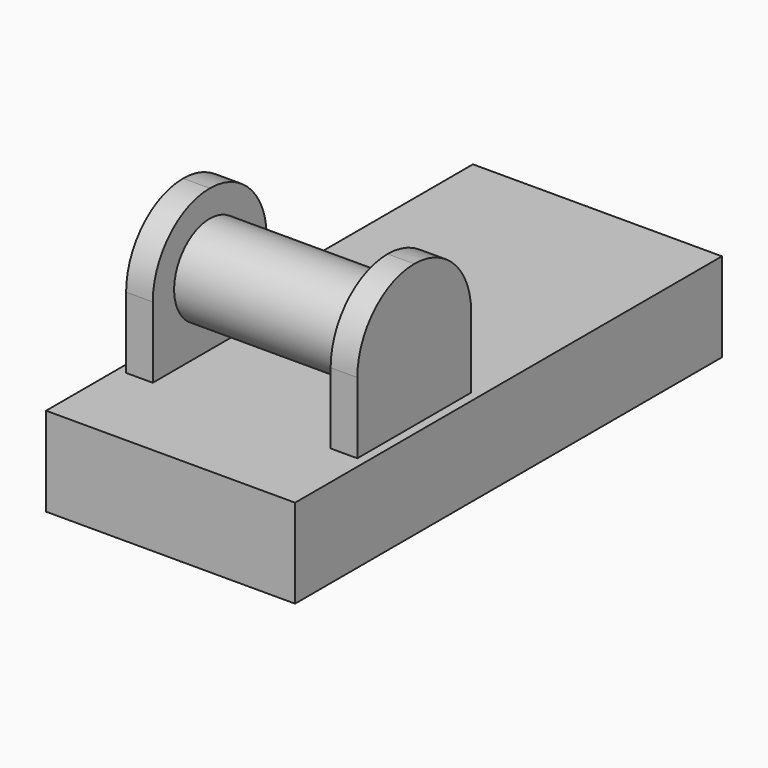
from build123d import *

# Parameters (mm, degrees)
F1_DEPTH = 30
F3_W     = 1.5
F3_H     = 8
F4_DEPTH = 8
F5_R     = 2.5
F6_DEPTH = 13
F7_R     = 3.99999


# Not quite as in the source:
# - a fillet or chamfer is up to 0.001 mm smaller than in the source, because OpenCascade refuses the exact size


with BuildPart() as f1:
    # F0 (on Front) → F1 (new body)
    with BuildSketch(Plane.XZ):
        Polygon((-14, 0), (0, 0), (0, 5), (-0.5, 5), (-2, 5), (-12, 5), (-13.5, 5), (-14, 5), align=None)
    extrude(amount=F1_DEPTH)

    # F3 (on offset) → F4 (join)
    with BuildSketch(Plane.XZ.offset(25)):
        with Locations((-12.75, 9)):
            Rectangle(F3_W, F3_H)
        with Locations((-1.25, 9)):
            Rectangle(F3_W, F3_H)
    extrude(amount=-F4_DEPTH)

    # F5 (on face) → F6 (join, through all)
    with BuildSketch(Plane.YZ.offset(-0.5)):
        with Locations((-21, 9)):
            Circle(F5_R)
    extrude(amount=-F6_DEPTH)

    # F7 (radius 4 in the source; OpenCascade refuses exactly that, so slightly less here)
    f7_edges = [f1.edges().sort_by_distance(p)[0] for p in [
        (-1.25, -17, 13),
        (-1.25, -25, 13),
        (-12.75, -17, 13),
        (-12.75, -25, 13),
    ]]
    fillet(f7_edges, radius=F7_R)


solid = f1.part
